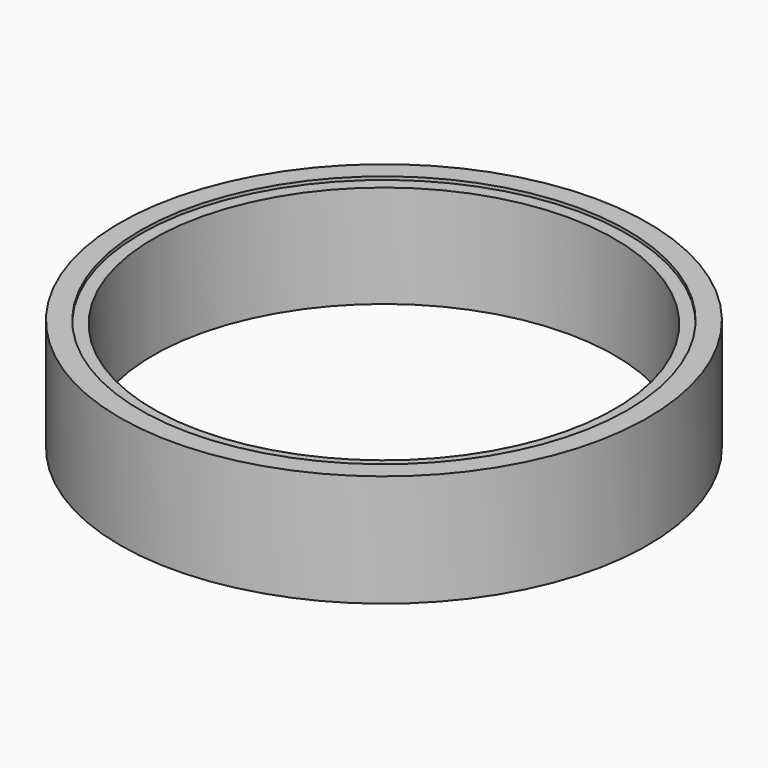
from build123d import *

# Parameters (mm, degrees)
F7_W     = 50.8
F7_H     = 12.7
F8_DEPTH = 130.811


# Not quite as in the source:
# - a feature of the source that left no trace in its solid (it failed there, or was rolled back) is left out


with BuildPart() as f1:
    # F0 (on Right) → F1 (revolve)
    with BuildSketch(Plane.YZ):
        with BuildLine():
            Line((-120.65, 3.175), (-114.3, 3.175))
            Line((-114.3, 3.175), (-114.3, 53.975))
            Line((-114.3, 53.975), (-120.65, 53.975))
            Line((-120.65, 53.975), (-120.65, 47.625))
            ThreePointArc((-120.65, 47.625), (-118.4049359697, 46.6950640303), (-117.475, 44.45))
            ThreePointArc((-117.475, 44.45), (-118.4049359697, 42.2049359697), (-120.65, 41.275))
            Line((-120.65, 41.275), (-120.65, 15.875))
            ThreePointArc((-120.65, 15.875), (-118.4049359697, 14.9450640303), (-117.475, 12.7))
            ThreePointArc((-117.475, 12.7), (-118.4049359697, 10.4549359697), (-120.65, 9.525))
            Line((-120.65, 9.525), (-120.65, 3.175))
        make_face()
    revolve(axis=Axis((0, 0, 81.893116076), (0, 0, 1)))


with BuildPart() as f3:
    # F2 (on Right) → F3 (revolve)
    with BuildSketch(Plane.YZ):
        with BuildLine():
            Line((130.81, 55.5625), (120.65, 55.5625))
            Line((120.65, 55.5625), (120.65, 47.625))
            ThreePointArc((120.65, 47.625), (122.8950640303, 46.6950640303), (123.825, 44.45))
            ThreePointArc((123.825, 44.45), (122.8950640303, 42.2049359697), (120.65, 41.275))
            Line((120.65, 41.275), (120.65, 15.875))
            ThreePointArc((120.65, 15.875), (122.8950640303, 14.9450640303), (123.825, 12.7))
            ThreePointArc((123.825, 12.7), (122.8950640303, 10.4549359697), (120.65, 9.525))
            Line((120.65, 9.525), (120.65, 0))
            Line((120.65, 0), (130.81, 0))
            Line((130.81, 0), (130.81, 55.5625))
        make_face()
    revolve(axis=Axis((0, 0, 8.8796737873), (0, 0, -1)))


with BuildPart() as f5:
    # F0 (on Right) → F5 (revolve)
    with BuildSketch(Plane.YZ):
        with BuildLine():
            Line((-120.65, 3.175), (-114.3, 3.175))
            Line((-114.3, 3.175), (-114.3, 53.975))
            Line((-114.3, 53.975), (-120.65, 53.975))
            Line((-120.65, 53.975), (-120.65, 47.625))
            ThreePointArc((-120.65, 47.625), (-118.4049359697, 46.6950640303), (-117.475, 44.45))
            ThreePointArc((-117.475, 44.45), (-118.4049359697, 42.2049359697), (-120.65, 41.275))
            Line((-120.65, 41.275), (-120.65, 15.875))
            ThreePointArc((-120.65, 15.875), (-118.4049359697, 14.9450640303), (-117.475, 12.7))
            ThreePointArc((-117.475, 12.7), (-118.4049359697, 10.4549359697), (-120.65, 9.525))
            Line((-120.65, 9.525), (-120.65, 3.175))
        make_face()
    revolve(axis=Axis((0, 0, 81.893116076), (0, 0, 1)))


with BuildPart() as f8_tool:
    # F7 (on Front) → F8 (new body, through all)
    with BuildSketch(Plane.XZ):
        with Locations((0, 28.575)):
            Rectangle(F7_W, F7_H)
    extrude(amount=F8_DEPTH)


with BuildPart() as f1_1:
    add(f1.part)

    # F8: cut by f8_tool
    add(f8_tool.part, mode=Mode.SUBTRACT)


with BuildPart() as f5_1:
    add(f5.part)

    # F8: cut by f8_tool
    add(f8_tool.part, mode=Mode.SUBTRACT)


with BuildPart() as f9:
    # F0 (on Right) → F9 (revolve)
    with BuildSketch(Plane.YZ):
        with BuildLine():
            ThreePointArc((-120.65, 15.875), (-123.825, 12.7), (-120.65, 9.525))
            Line((-120.65, 9.525), (-120.65, 15.875))
        make_face()
        with BuildLine():
            Line((-120.65, 15.875), (-120.65, 9.525))
            ThreePointArc((-120.65, 9.525), (-118.4049359697, 10.4549359697), (-117.475, 12.7))
            ThreePointArc((-117.475, 12.7), (-118.4049359697, 14.9450640303), (-120.65, 15.875))
        make_face()
    revolve(axis=Axis((0, 0, 81.893116076), (0, 0, 1)))


solid = Compound([f3.part, f1_1.part, f9.part])
